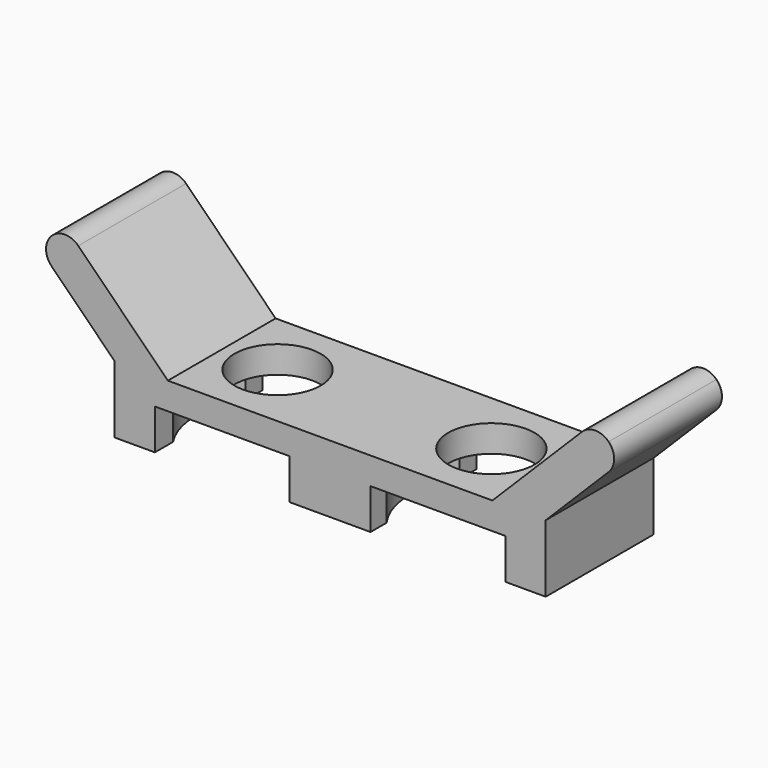
from build123d import *

# Parameters (mm, degrees)
F1_DEPTH = 4.7625
F2_R     = 5.08
F3_DEPTH = 3.175
F6_DEPTH = 15.875
F7_R     = 2.22249


# Not quite as in the source:
# - a fillet or chamfer is up to 0.001 mm smaller than in the source, because OpenCascade refuses the exact size


with BuildPart() as f1:
    # F0 (on Top) → F1 (new body)
    with BuildSketch(Plane.XY):
        with BuildLine():
            Line((0, 15.875), (0, 0))
            Line((0, 0), (4.7625, 0))
            Line((4.7625, 0), (4.7625, 2.6723581453))
            ThreePointArc((4.7625, 2.6723581453), (3.1538333333, 8.0077018914), (4.7625, 13.3430456375))
            Line((4.7625, 13.3430456375), (4.7625, 15.875))
            Line((4.7625, 15.875), (3.175, 15.875))
            Line((3.175, 15.875), (0, 15.875))
        make_face()
    extrude(amount=F1_DEPTH)


with BuildPart() as f1b:
    # F0 (on Top) → F1, piece 2 (new body)
    with BuildSketch(Plane.XY):
        with BuildLine():
            Line((20.6375, 2.3662392068), (20.6375, 0))
            Line((20.6375, 0), (25.4, 0))
            Line((25.4, 0), (25.4, 15.875))
            Line((25.4, 15.875), (20.8491666667, 15.875))
            Line((20.8491666667, 15.875), (20.8491666667, 13.3430456375))
            ThreePointArc((20.8491666667, 13.3430456375), (22.4560393469, 7.8216161703), (20.6375, 2.3662392068))
        make_face()
        with BuildLine():
            Line((25.4, 15.875), (25.4, 0))
            Line((25.4, 0), (30.1625, 0))
            Line((30.1625, 0), (30.1625, 2.3662392068))
            ThreePointArc((30.1625, 2.3662392068), (28.3439606531, 7.8216161703), (29.9508333333, 13.3430456375))
            Line((29.9508333333, 13.3430456375), (29.9508333333, 15.875))
            Line((29.9508333333, 15.875), (25.4, 15.875))
        make_face()
    extrude(amount=F1_DEPTH)


with BuildPart() as f1c:
    # F0 (on Top) → F1, piece 3 (new body)
    with BuildSketch(Plane.XY):
        with BuildLine():
            Line((46.0375, 2.6723581453), (46.0375, 0))
            Line((46.0375, 0), (50.8, 0))
            Line((50.8, 0), (50.8, 15.875))
            Line((50.8, 15.875), (46.0375, 15.875))
            Line((46.0375, 15.875), (46.0375, 13.3430456375))
            ThreePointArc((46.0375, 13.3430456375), (47.6461666667, 8.0077018914), (46.0375, 2.6723581453))
        make_face()
    extrude(amount=F1_DEPTH)


with BuildPart() as f3:
    # F2 (on face) → F3 (new body)
    with BuildSketch(Plane.XY.offset(4.7625)):
        with BuildLine():
            Line((25.4, 15.875), (4.7625, 15.875))
            Line((4.7625, 15.875), (4.7625, 13.3430456375))
            ThreePointArc((4.7625, 13.3430456375), (3.1538333333, 8.0077018914), (4.7625, 2.6723581453))
            Line((4.7625, 2.6723581453), (4.7625, 0))
            Line((4.7625, 0), (20.6375, 0))
            Line((20.6375, 0), (25.4, 0))
            Line((25.4, 0), (25.4, 2.2267585155))
            Line((25.4, 2.2267585155), (25.4, 15.875))
        make_face()
        with Locations((12.8058333333, 8.0077018914)):
            Circle(F2_R, mode=Mode.SUBTRACT)
        Polygon((46.0375, 15.875), (25.4, 15.875), (25.4, 2.2267585155), (25.4, 0), (30.1625, 0), (50.8, 0), (50.8, 15.875), align=None)
        with Locations((37.9941666667, 8.0077018914)):
            Circle(F2_R, mode=Mode.SUBTRACT)
        with BuildLine():
            Line((4.7625, 15.875), (0, 15.875))
            Line((0, 15.875), (0, 0))
            Line((0, 0), (4.7625, 0))
            Line((4.7625, 0), (4.7625, 2.6723581453))
            ThreePointArc((4.7625, 2.6723581453), (3.1538333333, 8.0077018914), (4.7625, 13.3430456375))
            Line((4.7625, 13.3430456375), (4.7625, 15.875))
        make_face()
    extrude(amount=F3_DEPTH)


with BuildPart() as f1_1:
    add(f1.part)

    # F4: union F3, F1b, F1c
    add(f3.part)
    add(f1b.part)
    add(f1c.part)

    # F5 (on face) → F6 (join)
    with BuildSketch(Plane.XZ):
        Polygon((56.6371664787, 20.0608457634), (44.5138207153, 7.9375), (50.8, 7.9375), (59.7802561211, 16.9177561211), align=None)
        Polygon((-8.9802561211, 16.9177561211), (0, 7.9375), (6.2861792847, 7.9375), (-5.8371664787, 20.0608457634), align=None)
    extrude(amount=-F6_DEPTH)

    # F7 (radius 2.2225 in the source; OpenCascade refuses exactly that, so slightly less here)
    f7_edges = [f1_1.edges().sort_by_distance(p)[0] for p in [
        (-8.980256, 7.9375, 16.917756),
        (-5.837166, 7.9375, 20.060846),
        (56.637166, 7.9375, 20.060846),
        (59.780256, 7.9375, 16.917756),
    ]]
    fillet(f7_edges, radius=F7_R)


solid = f1_1.part
